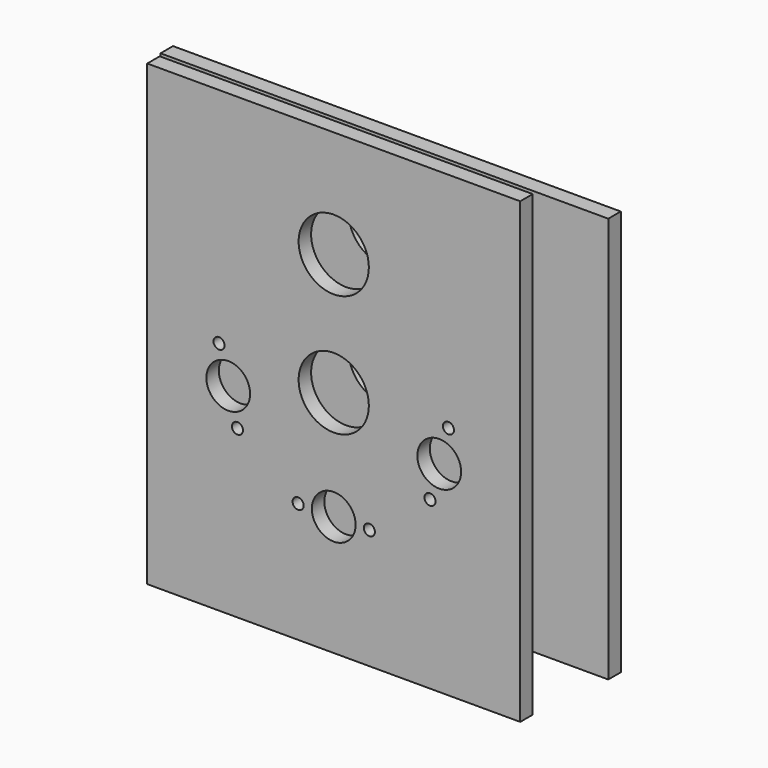
from build123d import *

# Parameters (mm, degrees)
F0_W     = 151.8040597439
F0_H     = 186.5415424109
F0_R     = 8.9027
F0_R_2   = 14.2875
F1_DEPTH = 6.35
F2_DEPTH = 6.351
F3_D     = 4.5
F5_W     = 182.2301670909
F5_H     = 165.1131734252
F5_R     = 14.2875
F6_DEPTH = 6.35


# Not quite as in the source:
# - a pattern or mirror of a feature is missing from the dataset's text; its kind, count and spacing are read off the source's solid


with BuildPart() as f1:
    # F0 (on Front) → F1 (new body)
    with BuildSketch(Plane.XZ):
        Rectangle(F0_W, F0_H)
        with Locations((0, -44.45)):
            Circle(F0_R, mode=Mode.SUBTRACT)
        Circle(F0_R_2, mode=Mode.SUBTRACT)
        with Locations((0, 49.53)):
            Circle(F0_R_2, mode=Mode.SUBTRACT)
        with Locations((0, -44.45)):
            Circle(F0_R)
    extrude(amount=F1_DEPTH)

    # F0 (on Front) → F2 (cut, through all)
    with BuildSketch(Plane.XZ):
        with Locations((0, -44.45)):
            Circle(F0_R)
    f2 = extrude(amount=F2_DEPTH, mode=Mode.SUBTRACT)

    # F2_copies: F2 across plane
    add(f2.mirror(Plane(origin=(0, 0, 0), x_dir=(-0.608761429, 0, -0.7933533403), z_dir=(-0.7933533403, 0, 0.608761429))), mode=Mode.SUBTRACT)

    # F2_copies1: F2 across plane
    add(f2.mirror(Plane(origin=(0, 0, 0), x_dir=(-0.608761429, 0, 0.7933533403), z_dir=(0.7933533403, 0, 0.608761429))), mode=Mode.SUBTRACT)

    # F3 (through all)
    with Locations(Plane(origin=(0, 0, 0), x_dir=(1, 0, 0), z_dir=(0, 1, 0))):
        with Locations((-14.5, 44.45), (14.5, 44.45)):
            f3 = Hole(F3_D / 2)

    # F3_copies: F3 across plane
    add(f3.mirror(Plane(origin=(0, 0, 0), x_dir=(-0.608761429, 0, -0.7933533403), z_dir=(-0.7933533403, 0, 0.608761429))), mode=Mode.SUBTRACT)

    # F3_copies1: F3 across plane
    add(f3.mirror(Plane(origin=(0, 0, 0), x_dir=(-0.608761429, 0, 0.7933533403), z_dir=(0.7933533403, 0, 0.608761429))), mode=Mode.SUBTRACT)


with BuildPart() as f6:
    # F5 (on offset) → F6 (new body)
    with BuildSketch(Plane.XZ.offset(-19.05)):
        with Locations((0.2993606031, -0.803668052)):
            Rectangle(F5_W, F5_H)
        Circle(F5_R, mode=Mode.SUBTRACT)
        with Locations((0, 49.53)):
            Circle(F5_R, mode=Mode.SUBTRACT)
    extrude(amount=-F6_DEPTH)


solid = Compound([f1.part, f6.part])
